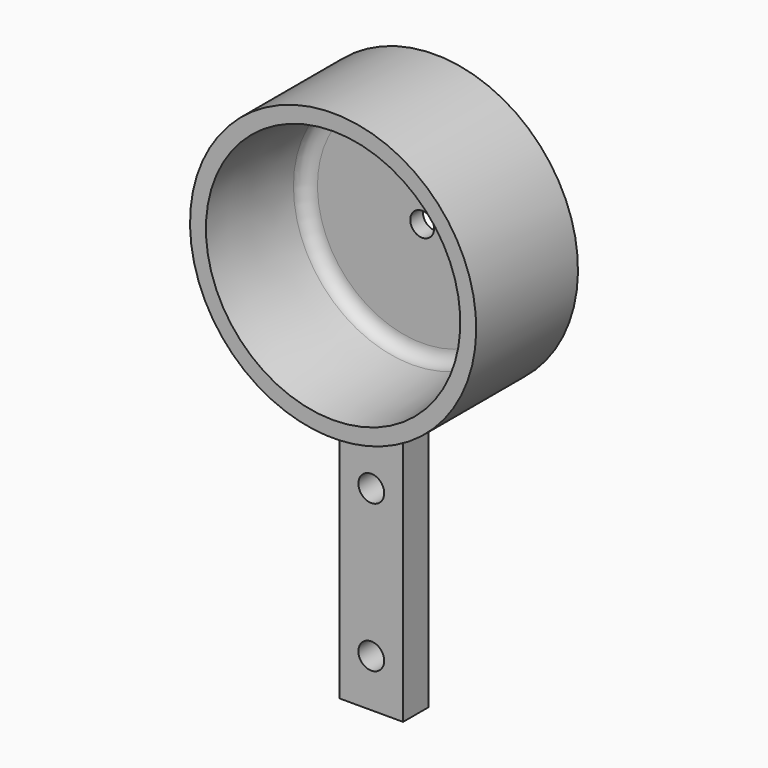
from build123d import *
from build123d import SkipClean  # not in build123d's __all__

# Parameters (mm, degrees)
F0_R     = 2.5781
F0_R_2   = 2.38125
F2_DEPTH = 25.4
F4_R     = 2.5781
F5_DEPTH = 9.525
F6_R     = 2.5781
F7_DEPTH = 9.525


with BuildPart() as f2:
    # F0 (on Front) → F2 (new body)
    with BuildSketch(Plane.XZ):
        with BuildLine():
            ThreePointArc((6.35, -31.4308964237), (7.2239350333, -28.6812657667), (9.525, -26.9407683632))
            ThreePointArc((9.525, -26.9407683632), (0, 28.575), (-9.525, -26.9407683632))
            ThreePointArc((-9.525, -26.9407683632), (-7.2239350333, -28.6812657667), (-6.35, -31.4308964237))
            Line((-6.35, -31.4308964237), (-6.35, -80.264))
            Line((-6.35, -80.264), (6.35, -80.264))
            Line((6.35, -80.264), (6.35, -31.4308964237))
        make_face()
        with Locations((0, -70.739)):
            Circle(F0_R, mode=Mode.SUBTRACT)
        with Locations((0, -41.275)):
            Circle(F0_R, mode=Mode.SUBTRACT)
        Circle(F0_R_2, mode=Mode.SUBTRACT)
    extrude(amount=-F2_DEPTH)

    # F1 (on Right) → F3 (revolve, cut)
    with BuildSketch(Plane.YZ):
        with BuildLine():
            Line((19.6890045478, 23.677435306), (0, 25.4))
            Line((0, 25.4), (0, 0))
            Line((0, 0), (22.225, 0))
            Line((22.225, 0), (22.225, 20.9098819103))
            ThreePointArc((22.225, 20.9098819103), (21.4951236013, 22.7867559559), (19.6890045478, 23.677435306))
        make_face()
    revolve(axis=Axis((0, 12.7, 0), (0, 1, 0)), mode=Mode.SUBTRACT)

    # F4 (on face) → F5 (cut)
    with BuildSketch(Plane.XZ):
        with BuildLine():
            ThreePointArc((9.525, -26.9407683632), (0, -28.575), (-9.525, -26.9407683632))
            ThreePointArc((-9.525, -26.9407683632), (-7.2239350333, -28.6812657667), (-6.35, -31.4308964237))
            Line((-6.35, -31.4308964237), (-6.35, -80.264))
            Line((-6.35, -80.264), (6.35, -80.264))
            Line((6.35, -80.264), (6.35, -31.4308964237))
            ThreePointArc((6.35, -31.4308964237), (7.2239350333, -28.6812657667), (9.525, -26.9407683632))
        make_face()
        with Locations((0, -70.739)):
            Circle(F4_R, mode=Mode.SUBTRACT)
        with Locations((0, -41.275)):
            Circle(F4_R, mode=Mode.SUBTRACT)
    with SkipClean():  # cleaning this boolean's faces spoils the solid; the shape is the same uncleaned
        extrude(amount=-F5_DEPTH, mode=Mode.SUBTRACT)

    # F6 (on face) → F7 (cut)
    with BuildSketch(Plane(origin=(0, 25.4, 0), x_dir=(-1, 0, 0), z_dir=(0, 1, 0))):
        with BuildLine():
            ThreePointArc((9.525, -26.9407683632), (0, -28.575), (-9.525, -26.9407683632))
            ThreePointArc((-9.525, -26.9407683632), (-7.2239350333, -28.6812657667), (-6.35, -31.4308964237))
            Line((-6.35, -31.4308964237), (-6.35, -80.264))
            Line((-6.35, -80.264), (6.35, -80.264))
            Line((6.35, -80.264), (6.35, -31.4308964237))
            ThreePointArc((6.35, -31.4308964237), (7.2239350333, -28.6812657667), (9.525, -26.9407683632))
        make_face()
        with Locations((0, -70.739)):
            Circle(F6_R, mode=Mode.SUBTRACT)
        with Locations((0, -41.275)):
            Circle(F6_R, mode=Mode.SUBTRACT)
    extrude(amount=-F7_DEPTH, mode=Mode.SUBTRACT)


solid = f2.part
